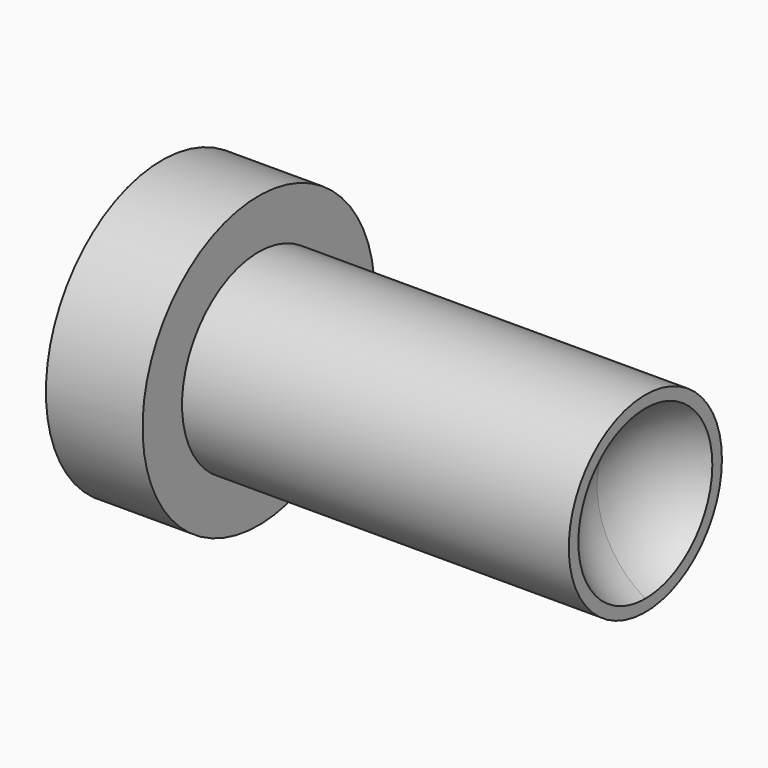
from build123d import *
from build123d import SkipClean  # not in build123d's __all__

# Parameters (mm, degrees)
F0_R     = 19.05
F1_DEPTH = 12.7
F2_R     = 12.573
F3_DEPTH = 50.8


with BuildPart() as f1:
    # F0 (on Right) → F1 (new body)
    with BuildSketch(Plane.YZ):
        Circle(F0_R)
    extrude(amount=F1_DEPTH)

    # F2 (on face) → F3 (join)
    with BuildSketch(Plane.YZ.offset(12.7)):
        Circle(F2_R)
    extrude(amount=F3_DEPTH)

    # F4 (on Front) → F5 (revolve, cut)
    with BuildSketch(Plane.XZ):
        with BuildLine():
            Line((69.85, -12.7), (69.85, 12.7))
            ThreePointArc((69.85, 12.7), (57.15, 0), (69.85, -12.7))
        make_face()
    with SkipClean():  # cleaning this boolean's faces spoils the solid; the shape is the same uncleaned
        revolve(axis=Axis((69.85, 0, 17.1570373535), (0, 0, 1)), mode=Mode.SUBTRACT)


solid = f1.part
